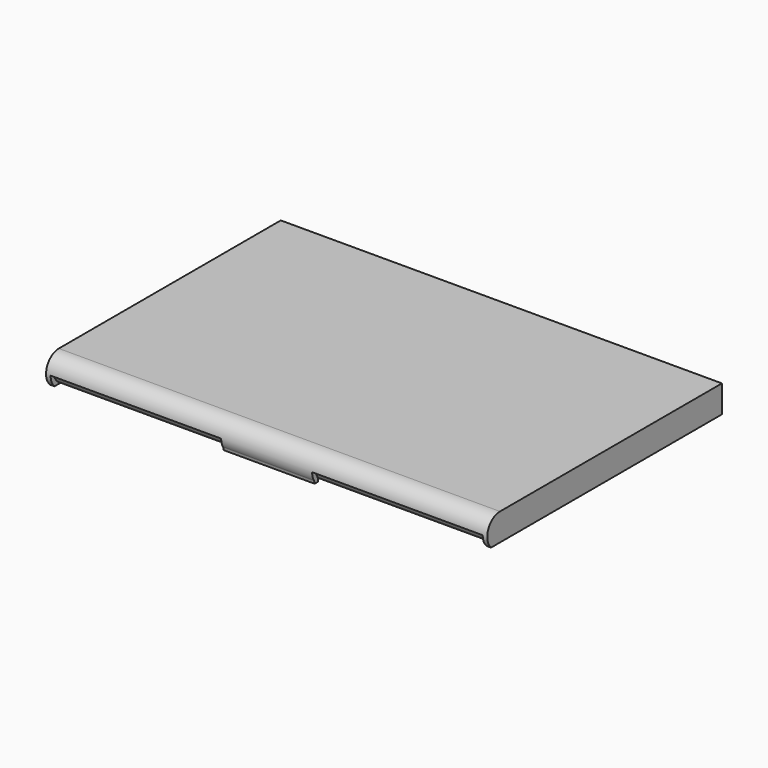
from build123d import *

# Parameters (mm, degrees)
F1_DEPTH       = 47.5
F2_T           = 1
F3_W           = 15
F3_H           = 1
F4_DEPTH       = 46.5
F4_DEPTH_BACK  = 46.5
F6_DEPTH       = 47.5
F6_DEPTH_BACK  = 47.5
F7_R           = 0.55
F8_DEPTH       = 1
F9_R           = 0.5
F10_DEPTH      = 1
F12_DEPTH      = 48.5
F13_T          = 1
F15_W          = 37.5
F15_H          = 10.6723425663
F16_DEPTH      = 144
F18_DEPTH      = 20
F20_DEPTH      = 20
F21_W          = 1
F21_H          = 2.9
F22_DEPTH      = 48.5
F22_DEPTH_BACK = 48.5
F23_R          = 0.45
F24_DEPTH      = 1.2
F25_R          = 0.45
F26_DEPTH      = 1.2


# Not quite as in the source:
# - an extrude ends at something that could not be found from the text; its depth is read off the source's solid
# - ends of sketch curves that miss each other by under 0.0002 mm in the source are joined
# - a shell that OpenCascade refuses in one call is made with other operations: the cavity is built on its own and cut out


with BuildPart() as f1:
    # F0 (on Right) → F1 (new body, symmetric)
    with BuildSketch(Plane.YZ):
        with BuildLine():
            Line((30, 2.5), (-30, 2.5))
            ThreePointArc((-30, 2.5), (-32.5, 0), (-30, -2.5))
            Line((-30, -2.5), (30, -2.5))
            Line((30, -2.5), (30, 2.5))
        make_face()
    extrude(amount=F1_DEPTH, both=True)

    # F2: shell of thickness 1, made by hand


with BuildPart() as f2_core1:
    # F2_t2: copy of F1
    add(f1.part)

    # the walls: a layer under each face that stays
    f2_faces = [f2_core1.faces().sort_by_distance(p)[0] for p in [
        (0, 0, -2.5),
        (47.5, -1.25, 0),
        (0, -32.5, 0),
        (-47.5, -1.25, 0),
    ]]
    thicken(f2_faces, amount=-F2_T, mode=Mode.SUBTRACT)


with BuildPart() as f1_1:
    add(f1.part)

    # what is left inside the walls is the cavity
    f2_cavity = [f2_core1.part.solids().sort_by_distance(p)[0] for p in [
        (-15.5, 0, 2.49),
    ]]
    add(f2_cavity, mode=Mode.SUBTRACT)

    # F3 (on Right) → F4 (join, two sides)
    with BuildSketch(Plane.YZ) as f4_sk:
        with Locations((-22.5, 2)):
            Rectangle(F3_W, F3_H)
    extrude(amount=F4_DEPTH)
    extrude(f4_sk.sketch, amount=-F4_DEPTH_BACK)

    # F5 (on Right) → F6 (join, two sides)
    with BuildSketch(Plane.YZ) as f6_sk:
        with BuildLine():
            Line((28.5, -2.5), (29.9848040611, -2.5))
            ThreePointArc((29.9848040611, -2.5), (29.9924019331, -2.4999807563), (30, -2.5))
            Line((30, -2.5), (30, 0.5))
            Line((30, 0.5), (28.5, 0.5))
            Line((28.5, 0.5), (28.5, -2.5))
        make_face()
        with BuildLine():
            Line((30, 0.5), (30, -2.5))
            ThreePointArc((30, -2.5), (31.5, -1), (30, 0.5))
        make_face()
    extrude(amount=F6_DEPTH)
    extrude(f6_sk.sketch, amount=-F6_DEPTH_BACK)

    # F7 (on face) → F8 (cut)
    with BuildSketch(Plane.YZ.offset(47.5)):
        with Locations((30, -1)):
            Circle(F7_R)
    extrude(amount=-F8_DEPTH, mode=Mode.SUBTRACT)

    # F9 (on face) → F10 (cut)
    with BuildSketch(Plane(origin=(-47.5, 0, 0), x_dir=(0, -1, 0), z_dir=(-1, 0, 0))):
        with Locations((-30, -1)):
            Circle(F9_R)
    extrude(amount=-F10_DEPTH, mode=Mode.SUBTRACT)


with BuildPart() as f12:
    # F11 (on Right) → F12 (new body, symmetric)
    with BuildSketch(Plane.YZ):
        with BuildLine():
            Line((31, 3.5), (-30, 3.5))
            ThreePointArc((-30, 3.5), (-33.2403703492, 1.3228756555), (-32.4494897428, -2.5))
            Line((-32.4494897428, -2.5), (-30, -2.5))
            Line((-30, -2.5), (31, -2.5))
            Line((31, -2.5), (31, 3.5))
        make_face()
    extrude(amount=F12_DEPTH, both=True)

    # F13: shell of thickness 1, made by hand


with BuildPart() as f13_core1:
    # F13_t2: copy of F12
    add(f12.part)

    # the walls: a layer under each face that stays
    f13_faces = [f13_core1.faces().sort_by_distance(p)[0] for p in [
        (0, 0.5, 3.5),
        (48.5, -1.25, 0.5),
        (0, -33.2403703492, 1.3228756555),
        (-48.5, -1.25, 0.5),
    ]]
    thicken(f13_faces, amount=-F13_T, mode=Mode.SUBTRACT)


with BuildPart() as f12_1:
    add(f12.part)

    # what is left inside the walls is the cavity
    f13_cavity = [f13_core1.part.solids().sort_by_distance(p)[0] for p in [
        (-15.833333, -0.724745, -2.49),
    ]]
    add(f13_cavity, mode=Mode.SUBTRACT)

    # F15 (on offset) → F16 (cut, through all)
    with BuildSketch(Plane.XZ.offset(30)):
        with Locations((-28.75, -5.3361712831)):
            Rectangle(F15_W, F15_H)
        with Locations((28.75, -5.3361712831)):
            Rectangle(F15_W, F15_H)
    extrude(amount=F16_DEPTH, mode=Mode.SUBTRACT)

    # F17 (on face) → F18 (cut, through all)
    with BuildSketch(Plane.YZ.offset(10)):
        with BuildLine():
            Line((-32.1650635095, -1.25), (-33.0310889132, -1.75))
            ThreePointArc((-33.0310889132, -1.75), (-32.7658290983, -2.1448052123), (-32.4494897428, -2.5))
            Line((-32.4494897428, -2.5), (-30, -2.5))
            ThreePointArc((-30, -2.5), (-31.25, -2.1650635095), (-32.1650635095, -1.25))
        make_face()
    extrude(amount=-F18_DEPTH, mode=Mode.SUBTRACT)

    # F19 (on face) → F20 (join, through all)
    with BuildSketch(Plane.YZ.offset(10)):
        with BuildLine():
            ThreePointArc((-33.0310889132, -1.75), (-32.8812382795, -2.1117714323), (-32.8301270189, -2.5))
            Line((-32.8301270189, -2.5), (-31.8301270189, -2.5))
            ThreePointArc((-31.8301270189, -2.5), (-31.9153124532, -1.8529523872), (-32.1650635095, -1.25))
            Line((-32.1650635095, -1.25), (-33.0310889132, -1.75))
        make_face()
    extrude(amount=-F20_DEPTH)

    # F21 (on Right) → F22 (join, two sides)
    with BuildSketch(Plane.YZ) as f22_sk:
        with Locations((30.5, 2.05)):
            Rectangle(F21_W, F21_H)
    extrude(amount=F22_DEPTH)
    extrude(f22_sk.sketch, amount=-F22_DEPTH_BACK)

    # F23 (on face) → F24 (join)
    with BuildSketch(Plane.YZ.offset(-47.5)):
        with Locations((30, -1)):
            Circle(F23_R)
    extrude(amount=F24_DEPTH)

    # F25 (on face) → F26 (join)
    with BuildSketch(Plane(origin=(47.5, 0, 0), x_dir=(0, -1, 0), z_dir=(-1, 0, 0))):
        with Locations((-30, -1)):
            Circle(F25_R)
    extrude(amount=F26_DEPTH)


solid = Compound([f1_1.part, f12_1.part])
